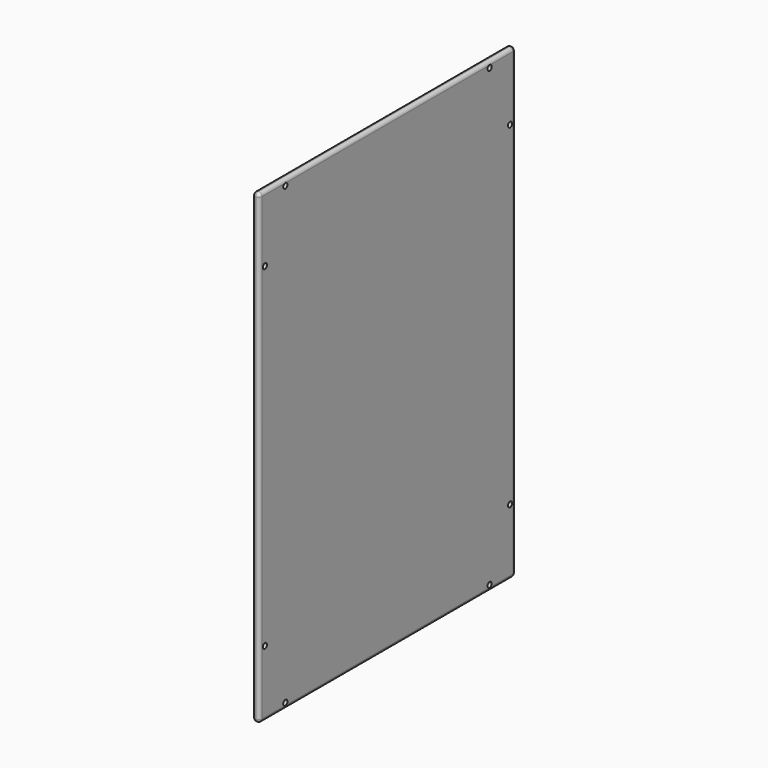
from build123d import *

# Parameters (mm, degrees)
F0_W         = 438.15
F0_H         = 638.175
F1_DEPTH     = 9.525
F3_D         = 7.14375
F4_T1_DEPTH  = 628.6480686291
F4_T3_DEPTH  = 428.6230686291
F4_S7_W      = 5.2402522539
F4_S7_H      = 5.2402522539
F4_T8_DEPTH  = 5.240252254
F4_S13_W     = 5.2402522539
F4_S13_H     = 5.2402522539
F4_T14_DEPTH = 5.240252254
F4_S19_W     = 5.2402522539
F4_S19_H     = 5.2402522539
F4_T20_DEPTH = 5.240252254
F4_S25_W     = 5.2402522539
F4_S25_H     = 5.2402522539
F4_T26_DEPTH = 5.240252254
F4_S31_W     = 5.2402522539
F4_S31_H     = 5.2402522539
F4_T32_DEPTH = 5.240252254
F4_S37_W     = 5.2402522539
F4_S37_H     = 5.2402522539
F4_T38_DEPTH = 5.240252254
F4_S43_W     = 5.2402522539
F4_S43_H     = 5.2402522539
F4_T44_DEPTH = 5.240252254
F4_S49_W     = 5.2402522539
F4_S49_H     = 5.2402522539
F4_T50_DEPTH = 5.240252254


# Not quite as in the source:
# - a fillet or chamfer that OpenCascade refuses, or shapes differently, is made with other operations: its cross-section is extruded or revolved along the edge and cut away or added


with BuildPart() as f1:
    # F0 (on Right) → F1 (new body)
    with BuildSketch(Plane.YZ):
        Rectangle(F0_W, F0_H)
    extrude(amount=F1_DEPTH)

    # F3 (through all)
    with Locations(Plane.YZ.offset(9.525)):
        with Locations((-174.625, 311.15), (-209.55, 228.6), (-209.55, -228.6), (-174.625, -311.15), (174.625, -311.15), (209.55, -228.6), (174.625, 311.15), (209.55, 228.6)):
            Hole(F3_D / 2)

    # F4: fillet of radius 4.7625 on 12 edges, made by hand

    # F4_s2 → F4_t1 (cut)
    with BuildSketch(Plane.XY.offset(-314.3240343146)):
        with BuildLine():
            ThreePointArc((4.7634656854, -219.0754), (1.3949039546, -217.6800960454), (-0.0004, -214.3115343146))
            Line((-0.0004, -214.3115343146), (-0.4767865685, -214.3115343146))
            ThreePointArc((-0.4767865685, -214.3115343146), (-0.4763865685, -216.6932671573), (-0.4763865685, -219.075))
            Line((-0.4763865685, -219.075), (0, -219.5513865685))
            ThreePointArc((0, -219.5513865685), (2.3817328427, -219.5513865685), (4.7634656854, -219.5517865685))
            Line((4.7634656854, -219.5517865685), (4.7634656854, -219.0754))
        make_face()
        with BuildLine():
            ThreePointArc((4.7615343146, -219.0754), (8.1300960454, -217.6800960454), (9.5254, -214.3115343146))
            Line((9.5254, -214.3115343146), (10.0017865685, -214.3115343146))
            ThreePointArc((10.0017865685, -214.3115343146), (10.0013865685, -216.6932671573), (10.0013865685, -219.075))
            Line((10.0013865685, -219.075), (9.525, -219.5513865685))
            ThreePointArc((9.525, -219.5513865685), (7.1432671573, -219.5513865685), (4.7615343146, -219.5517865685))
            Line((4.7615343146, -219.5517865685), (4.7615343146, -219.0754))
        make_face()
        with BuildLine():
            ThreePointArc((4.7634656854, 219.0754), (1.3949039546, 217.6800960454), (-0.0004, 214.3115343146))
            Line((-0.0004, 214.3115343146), (-0.4767865685, 214.3115343146))
            ThreePointArc((-0.4767865685, 214.3115343146), (-0.4763865685, 216.6932671573), (-0.4763865685, 219.075))
            Line((-0.4763865685, 219.075), (0, 219.5513865685))
            ThreePointArc((0, 219.5513865685), (2.3817328427, 219.5513865685), (4.7634656854, 219.5517865685))
            Line((4.7634656854, 219.5517865685), (4.7634656854, 219.0754))
        make_face()
        with BuildLine():
            ThreePointArc((4.7615343146, 219.0754), (8.1300960454, 217.6800960454), (9.5254, 214.3115343146))
            Line((9.5254, 214.3115343146), (10.0017865685, 214.3115343146))
            ThreePointArc((10.0017865685, 214.3115343146), (10.0013865685, 216.6932671573), (10.0013865685, 219.075))
            Line((10.0013865685, 219.075), (9.525, 219.5513865685))
            ThreePointArc((9.525, 219.5513865685), (7.1432671573, 219.5513865685), (4.7615343146, 219.5517865685))
            Line((4.7615343146, 219.5517865685), (4.7615343146, 219.0754))
        make_face()
    extrude(amount=F4_T1_DEPTH, mode=Mode.SUBTRACT)

    # F4_s4 → F4_t3 (cut)
    with BuildSketch(Plane.XZ.offset(-214.3115343146)):
        with BuildLine():
            ThreePointArc((9.5254, 314.3240343146), (8.1300960454, 317.6925960454), (4.7615343146, 319.0879))
            Line((4.7615343146, 319.0879), (4.7615343146, 319.5642865685))
            ThreePointArc((4.7615343146, 319.5642865685), (7.1432671573, 319.5638865685), (9.525, 319.5638865685))
            Line((9.525, 319.5638865685), (10.0013865685, 319.0875))
            ThreePointArc((10.0013865685, 319.0875), (10.0013865685, 316.7057671573), (10.0017865685, 314.3240343146))
            Line((10.0017865685, 314.3240343146), (9.5254, 314.3240343146))
        make_face()
        with BuildLine():
            ThreePointArc((-0.0004, 314.3240343146), (1.3949039546, 317.6925960454), (4.7634656854, 319.0879))
            Line((4.7634656854, 319.0879), (4.7634656854, 319.5642865685))
            ThreePointArc((4.7634656854, 319.5642865685), (2.3817328427, 319.5638865685), (0, 319.5638865685))
            Line((0, 319.5638865685), (-0.4763865685, 319.0875))
            ThreePointArc((-0.4763865685, 319.0875), (-0.4763865685, 316.7057671573), (-0.4767865685, 314.3240343146))
            Line((-0.4767865685, 314.3240343146), (-0.0004, 314.3240343146))
        make_face()
        with BuildLine():
            ThreePointArc((4.7634656854, -319.0879), (1.3949039546, -317.6925960454), (-0.0004, -314.3240343146))
            Line((-0.0004, -314.3240343146), (-0.4767865685, -314.3240343146))
            ThreePointArc((-0.4767865685, -314.3240343146), (-0.4763865685, -316.7057671573), (-0.4763865685, -319.0875))
            Line((-0.4763865685, -319.0875), (0, -319.5638865685))
            ThreePointArc((0, -319.5638865685), (2.3817328427, -319.5638865685), (4.7634656854, -319.5642865685))
            Line((4.7634656854, -319.5642865685), (4.7634656854, -319.0879))
        make_face()
        with BuildLine():
            ThreePointArc((4.7615343146, -319.0879), (8.1300960454, -317.6925960454), (9.5254, -314.3240343146))
            Line((9.5254, -314.3240343146), (10.0017865685, -314.3240343146))
            ThreePointArc((10.0017865685, -314.3240343146), (10.0013865685, -316.7057671573), (10.0013865685, -319.0875))
            Line((10.0013865685, -319.0875), (9.525, -319.5638865685))
            ThreePointArc((9.525, -319.5638865685), (7.1432671573, -319.5638865685), (4.7615343146, -319.5642865685))
            Line((4.7615343146, -319.5642865685), (4.7615343146, -319.0879))
        make_face()
    extrude(amount=F4_T3_DEPTH, mode=Mode.SUBTRACT)


with BuildPart() as f4_tool6:
    # F4_s7 → F4_t8 (new body)
    with BuildSketch(Plane.XZ.offset(214.3115343146)):
        with Locations((2.1433395585, 316.9441604416)):
            Rectangle(F4_S7_W, F4_S7_H)
    extrude(amount=F4_T8_DEPTH)

    # F4_s9 → F4_t10 (revolve, cut)
    with BuildSketch(Plane(origin=(4.7634656854, -214.3115343146, 314.3240343146), x_dir=(0.7071067812, 0, -0.7071067812), z_dir=(-0.7071067812, 0, -0.7071067812))):
        with BuildLine():
            ThreePointArc((0, -4.7638656854), (4.7638656854, 0), (0, 4.7638656854))
            Line((0, 4.7638656854), (0, -4.7638656854))
        make_face()
    revolve(axis=Axis((4.7634656854, -214.3115343146, 314.3240343146), (0, -1, 0)), mode=Mode.SUBTRACT)


with BuildPart() as f1_1:
    add(f1.part)

    # F4_t5: cut F4_tool6
    add(f4_tool6.part, mode=Mode.SUBTRACT)


with BuildPart() as f4_tool12:
    # F4_s13 → F4_t14 (new body)
    with BuildSketch(Plane.XY.offset(-314.3240343146)):
        with Locations((2.1433395585, -216.9316604416)):
            Rectangle(F4_S13_W, F4_S13_H)
    extrude(amount=-F4_T14_DEPTH)

    # F4_s15 → F4_t16 (revolve, cut)
    with BuildSketch(Plane(origin=(4.7634656854, -214.3115343146, -314.3240343146), x_dir=(0.7071067812, 0.7071067812, 0), z_dir=(-0.7071067812, 0.7071067812, 0))):
        with BuildLine():
            ThreePointArc((0, -4.7638656854), (4.7638656854, 0), (0, 4.7638656854))
            Line((0, 4.7638656854), (0, -4.7638656854))
        make_face()
    revolve(axis=Axis((4.7634656854, -214.3115343146, -314.3240343146), (0, 0, -1)), mode=Mode.SUBTRACT)


with BuildPart() as f1_2:
    add(f1_1.part)

    # F4_t11: cut F4_tool12
    add(f4_tool12.part, mode=Mode.SUBTRACT)


with BuildPart() as f4_tool18:
    # F4_s19 → F4_t20 (new body)
    with BuildSketch(Plane.XZ.offset(214.3115343146)):
        with Locations((7.3816604416, 316.9441604416)):
            Rectangle(F4_S19_W, F4_S19_H)
    extrude(amount=F4_T20_DEPTH)

    # F4_s21 → F4_t22 (revolve, cut)
    with BuildSketch(Plane(origin=(4.7615343146, -214.3115343146, 314.3240343146), x_dir=(-0.7071067812, 0, -0.7071067812), z_dir=(-0.7071067812, 0, 0.7071067812))):
        with BuildLine():
            ThreePointArc((0, -4.7638656854), (4.7638656854, 0), (0, 4.7638656854))
            Line((0, 4.7638656854), (0, -4.7638656854))
        make_face()
    revolve(axis=Axis((4.7615343146, -214.3115343146, 314.3240343146), (0, -1, 0)), mode=Mode.SUBTRACT)


with BuildPart() as f1_3:
    add(f1_2.part)

    # F4_t17: cut F4_tool18
    add(f4_tool18.part, mode=Mode.SUBTRACT)


with BuildPart() as f4_tool24:
    # F4_s25 → F4_t26 (new body)
    with BuildSketch(Plane.XY.offset(-314.3240343146)):
        with Locations((7.3816604416, -216.9316604416)):
            Rectangle(F4_S25_W, F4_S25_H)
    extrude(amount=-F4_T26_DEPTH)

    # F4_s27 → F4_t28 (revolve, cut)
    with BuildSketch(Plane(origin=(4.7615343146, -214.3115343146, -314.3240343146), x_dir=(-0.7071067812, 0.7071067812, 0), z_dir=(-0.7071067812, -0.7071067812, 0))):
        with BuildLine():
            ThreePointArc((0, -4.7638656854), (4.7638656854, 0), (0, 4.7638656854))
            Line((0, 4.7638656854), (0, -4.7638656854))
        make_face()
    revolve(axis=Axis((4.7615343146, -214.3115343146, -314.3240343146), (0, 0, -1)), mode=Mode.SUBTRACT)


with BuildPart() as f1_4:
    add(f1_3.part)

    # F4_t23: cut F4_tool24
    add(f4_tool24.part, mode=Mode.SUBTRACT)


with BuildPart() as f4_tool30:
    # F4_s31 → F4_t32 (new body)
    with BuildSketch(Plane.XZ.offset(-214.3115343146)):
        with Locations((7.3816604416, 316.9441604416)):
            Rectangle(F4_S31_W, F4_S31_H)
    extrude(amount=-F4_T32_DEPTH)

    # F4_s33 → F4_t34 (revolve, cut)
    with BuildSketch(Plane(origin=(4.7615343146, 214.3115343146, 314.3240343146), x_dir=(-0.7071067812, 0, -0.7071067812), z_dir=(0.7071067812, 0, -0.7071067812))):
        with BuildLine():
            ThreePointArc((0, -4.7638656854), (4.7638656854, 0), (0, 4.7638656854))
            Line((0, 4.7638656854), (0, -4.7638656854))
        make_face()
    revolve(axis=Axis((4.7615343146, 214.3115343146, 314.3240343146), (0, 1, 0)), mode=Mode.SUBTRACT)


with BuildPart() as f1_5:
    add(f1_4.part)

    # F4_t29: cut F4_tool30
    add(f4_tool30.part, mode=Mode.SUBTRACT)


with BuildPart() as f4_tool36:
    # F4_s37 → F4_t38 (new body)
    with BuildSketch(Plane.XZ.offset(-214.3115343146)):
        with Locations((2.1433395585, 316.9441604416)):
            Rectangle(F4_S37_W, F4_S37_H)
    extrude(amount=-F4_T38_DEPTH)

    # F4_s39 → F4_t40 (revolve, cut)
    with BuildSketch(Plane(origin=(4.7634656854, 214.3115343146, 314.3240343146), x_dir=(0.7071067812, 0, -0.7071067812), z_dir=(0.7071067812, 0, 0.7071067812))):
        with BuildLine():
            ThreePointArc((0, -4.7638656854), (4.7638656854, 0), (0, 4.7638656854))
            Line((0, 4.7638656854), (0, -4.7638656854))
        make_face()
    revolve(axis=Axis((4.7634656854, 214.3115343146, 314.3240343146), (0, 1, 0)), mode=Mode.SUBTRACT)


with BuildPart() as f1_6:
    add(f1_5.part)

    # F4_t35: cut F4_tool36
    add(f4_tool36.part, mode=Mode.SUBTRACT)


with BuildPart() as f4_tool42:
    # F4_s43 → F4_t44 (new body)
    with BuildSketch(Plane.XY.offset(-314.3240343146)):
        with Locations((2.1433395585, 216.9316604416)):
            Rectangle(F4_S43_W, F4_S43_H)
    extrude(amount=-F4_T44_DEPTH)

    # F4_s45 → F4_t46 (revolve, cut)
    with BuildSketch(Plane(origin=(4.7634656854, 214.3115343146, -314.3240343146), x_dir=(0.7071067812, -0.7071067812, 0), z_dir=(0.7071067812, 0.7071067812, 0))):
        with BuildLine():
            ThreePointArc((0, -4.7638656854), (4.7638656854, 0), (0, 4.7638656854))
            Line((0, 4.7638656854), (0, -4.7638656854))
        make_face()
    revolve(axis=Axis((4.7634656854, 214.3115343146, -314.3240343146), (0, 0, -1)), mode=Mode.SUBTRACT)


with BuildPart() as f1_7:
    add(f1_6.part)

    # F4_t41: cut F4_tool42
    add(f4_tool42.part, mode=Mode.SUBTRACT)


with BuildPart() as f4_tool48:
    # F4_s49 → F4_t50 (new body)
    with BuildSketch(Plane.XY.offset(-314.3240343146)):
        with Locations((7.3816604416, 216.9316604416)):
            Rectangle(F4_S49_W, F4_S49_H)
    extrude(amount=-F4_T50_DEPTH)

    # F4_s51 → F4_t52 (revolve, cut)
    with BuildSketch(Plane(origin=(4.7615343146, 214.3115343146, -314.3240343146), x_dir=(-0.7071067812, -0.7071067812, 0), z_dir=(0.7071067812, -0.7071067812, 0))):
        with BuildLine():
            ThreePointArc((0, -4.7638656854), (4.7638656854, 0), (0, 4.7638656854))
            Line((0, 4.7638656854), (0, -4.7638656854))
        make_face()
    revolve(axis=Axis((4.7615343146, 214.3115343146, -314.3240343146), (0, 0, -1)), mode=Mode.SUBTRACT)


with BuildPart() as f1_8:
    add(f1_7.part)

    # F4_t47: cut F4_tool48
    add(f4_tool48.part, mode=Mode.SUBTRACT)


solid = f1_8.part
